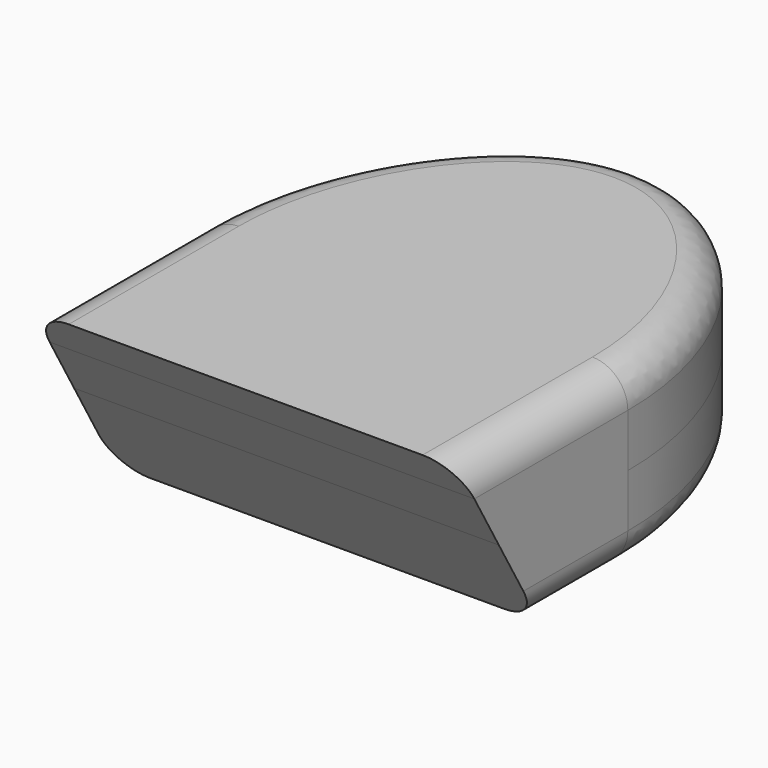
from build123d import *

# Parameters (mm, degrees)
F1_DEPTH = 12.5
F2_R     = 5
F4_DEPTH = 30


with BuildPart() as f1:
    # F0 (on Top) → F1 (new body, symmetric)
    with BuildSketch(Plane.XY):
        with BuildLine():
            Line((-30, 2.9789e-06), (-30, -30))
            Line((-30, -30), (0, -30))
            ThreePointArc((0, -30), (-21.2132044888, -21.2132023824), (-30, 2.9789e-06))
        make_face()
        with BuildLine():
            ThreePointArc((30, 0), (21.2132034356, -21.2132034356), (0, -30))
            Line((0, -30), (30, -30))
            Line((30, -30), (30, 0))
        make_face()
        with BuildLine():
            ThreePointArc((-30, 2.9789e-06), (-21.2132044888, -21.2132023824), (0, -30))
            ThreePointArc((0, -30), (21.2132034356, -21.2132034356), (30, 0))
            ThreePointArc((30, 0), (1.4895e-06, 30), (-30, 2.9789e-06))
        make_face()
        with BuildLine():
            add(Edge.make_bspline(
                [(0, 40), (-16.629870981, 40), (-30, 20.0504878896), (-30, 2.9789e-06)],
                knots=[0, 0, 0, 0, 49.9999976168, 49.9999976168, 49.9999976168, 49.9999976168], degree=3))
            ThreePointArc((-30, 2.9789e-06), (1.4895e-06, 30), (30, 0))
            add(Edge.make_bspline(
                [(0, 40), (16.629870981, 40), (30, 20.0504849106), (30, 0)],
                knots=[0, 0, 0, 0, 50, 50, 50, 50], degree=3))
        make_face()
    extrude(amount=F1_DEPTH, both=True)

    # F2
    f2_edges = [f1.edges().sort_by_distance(p)[0] for p in [
        (30, -15, -12.5),
        (30, -15, 12.5),
        (-30, -14.999999, 12.5),
        (-30, -14.999999, -12.5),
    ]]
    fillet(f2_edges, radius=F2_R)

    # F3 (on Right) → F4 (cut, symmetric)
    with BuildSketch(Plane.YZ):
        Polygon((-15.5662432703, -12.5), (-22.7831216351, 0), (-30, 0), (-30, -12.5), align=None)
        Polygon((-30, 0), (-22.7831216351, 0), (-27.1132486541, 7.5), (-30, 7.5), align=None)
        Polygon((-30, 7.5), (-27.1132486541, 7.5), (-30, 12.5), align=None)
    extrude(amount=F4_DEPTH, both=True, mode=Mode.SUBTRACT)


solid = f1.part
